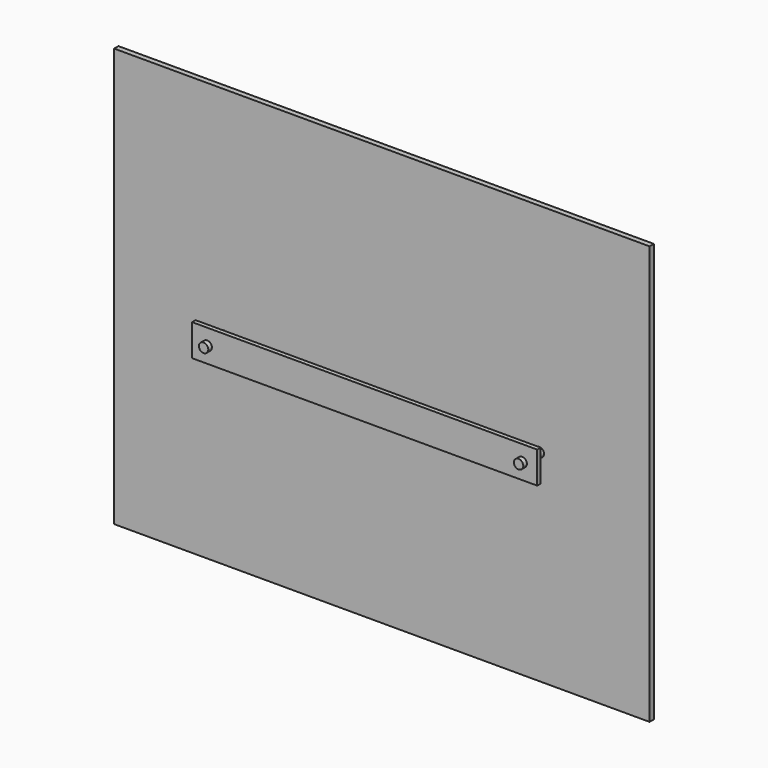
from build123d import *

# Parameters (mm, degrees)
F0_W          = 408.5518717766
F0_H          = 37.5892921885
F1_DEPTH      = 5.08
F3_DEPTH      = 5.334
F3_DEPTH_BACK = 25.4
F5_W          = 633.9019536972
F5_H          = 495.6407546997
F6_DEPTH      = 6.35


with BuildPart() as f1:
    # F0 (on Front) → F1 (new body)
    with BuildSketch(Plane.XZ):
        with Locations((0, -9.1188331868)):
            Rectangle(F0_W, F0_H)
    extrude(amount=F1_DEPTH)

    # F2 (on face) → F3 (join, two sides)
    with BuildSketch(Plane.XZ.offset(5.08)) as f3_sk:
        with BuildLine():
            ThreePointArc((-180.9181509954, -9.1188331868), (-186.4621341228, -3.5748500593), (-192.0061172503, -9.1188331868))
            Line((-192.0061172503, -9.1188331868), (-180.9181509954, -9.1188331868))
        make_face()
        with BuildLine():
            Line((-180.9181509954, -9.1188331868), (-192.0061172503, -9.1188331868))
            ThreePointArc((-192.0061172503, -9.1188331868), (-186.4621341228, -14.6628163142), (-180.9181509954, -9.1188331868))
        make_face()
    extrude(amount=F3_DEPTH)
    extrude(f3_sk.sketch, amount=-F3_DEPTH_BACK)

    # F4: F1 across plane


with BuildPart() as f1_1:
    add(f1.part)
    add(f1.part.mirror(Plane.YZ))


with BuildPart() as f6:
    # F5 (on face) → F6 (new body)
    with BuildSketch(Plane(origin=(0, 20.32, 0), x_dir=(-1, 0, 0), z_dir=(0, 1, 0))):
        Rectangle(F5_W, F5_H)
    extrude(amount=F6_DEPTH)


solid = Compound([f1_1.part, f6.part])
